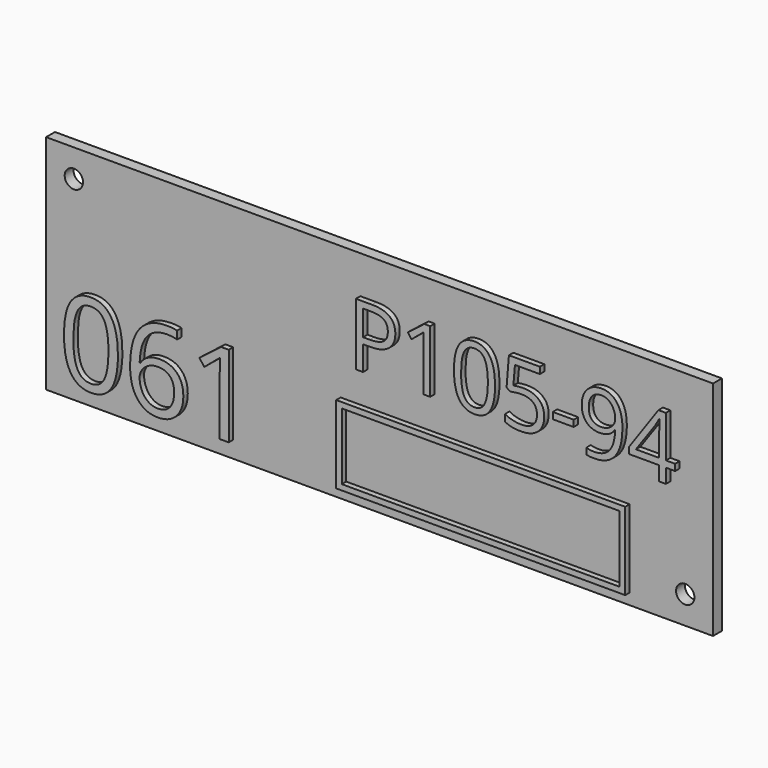
from build123d import *

# Parameters (mm, degrees)
F0_W         = 120
F0_H         = 40
F1_DEPTH     = 2
F3_D         = 3.3
F4_TEXT_SIZE = 15.6773087287
F5_DEPTH     = 1
F6_TEXT_SIZE = 20.5478077656
F7_DEPTH     = 1
F8_W         = 52
F8_H         = 14
F8_W_2       = 49.99999962
F8_H_2       = 11.99999962
F9_DEPTH     = 1


# Not quite as in the source:
# - Text() gives the source's letters only with a copy of the font that has no kerning and outlines rounded to 1/6400 em; it was checked with that copy


with BuildPart() as f1:
    # F0 (on Front) → F1 (new body)
    with BuildSketch(Plane.XZ):
        Rectangle(F0_W, F0_H)
    extrude(amount=F1_DEPTH)

    # F3 (through all)
    with Locations(Plane.XZ.offset(2)):
        with Locations((-55, 15), (55, -15)):
            Hole(F3_D / 2)

    # F4 (on face) → F5 (join)
    with BuildSketch(Plane.XZ.offset(2)):
        with Locations((-5, 2)):
            Text('P105-94', F4_TEXT_SIZE, font='Open Sans', text_align=(TextAlign.LEFT, TextAlign.BOTTOM))
    extrude(amount=F5_DEPTH)

    # F6 (on face) → F7 (join)
    with BuildSketch(Plane.XZ.offset(2)):
        with Locations((-57, -17)):
            Text('061', F6_TEXT_SIZE, font='Open Sans', text_align=(TextAlign.LEFT, TextAlign.BOTTOM))
    extrude(amount=F7_DEPTH)

    # F8 (on face) → F9 (join)
    with BuildSketch(Plane.XZ.offset(2)):
        with Locations((19, -11)):
            Rectangle(F8_W, F8_H)
        with Locations((19, -11)):
            Rectangle(F8_W_2, F8_H_2, mode=Mode.SUBTRACT)
    extrude(amount=F9_DEPTH)


solid = f1.part
